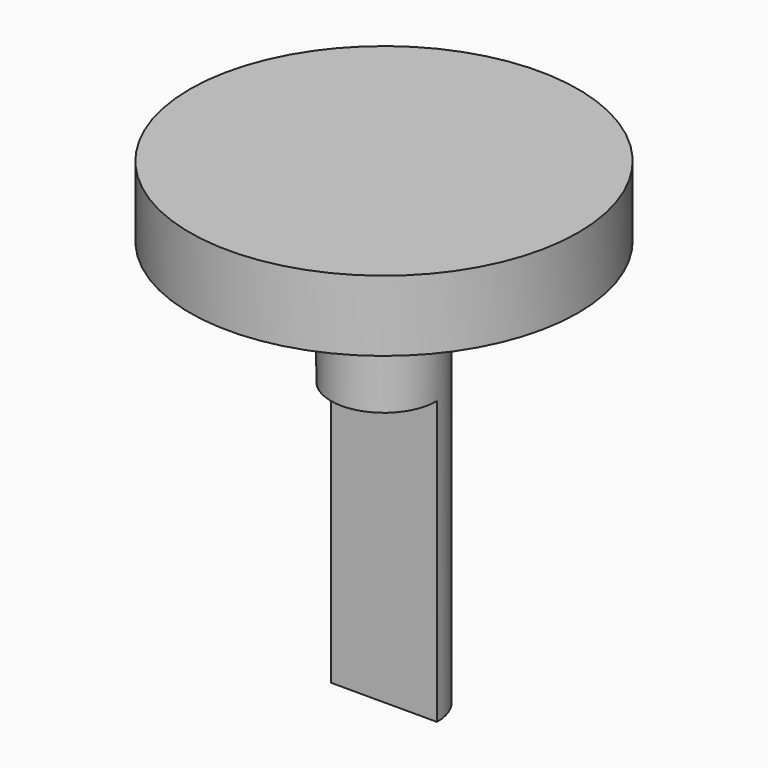
from build123d import *

# Parameters (mm, degrees)
F0_W     = 3
F0_H     = 7
F0_H_2   = 2
F0_H_3   = 16
F2_ANGLE = 180


# Not quite as in the source:
# - a feature names something its author has since deleted; it is built from what else it names


with BuildPart() as f1:
    # F0 (on Front) → F1 (revolve)
    with BuildSketch(Plane.XZ):
        Polygon((0, 14.5), (0, 12.5), (3, 12.5), (3, 10.5), (11, 10.5), (11, 14.5), align=None)
        with Locations((1.5, 7)):
            Rectangle(F0_W, F0_H)
        with Locations((1.5, 11.5)):
            Rectangle(F0_W, F0_H_2)
        with Locations((1.5, -4.5)):
            Rectangle(F0_W, F0_H_3)
    revolve(axis=Axis((0, 0, 1), (0, 0, -1)))

    # F0 (on Front) → F2 (revolve, cut)
    with BuildSketch(Plane.XZ):
        with Locations((-1.5, -4.5)):
            Rectangle(F0_W, F0_H_3)
    revolve(axis=Axis((0, 0, 1), (0, 0, 1)), revolution_arc=F2_ANGLE, mode=Mode.SUBTRACT)


solid = f1.part
